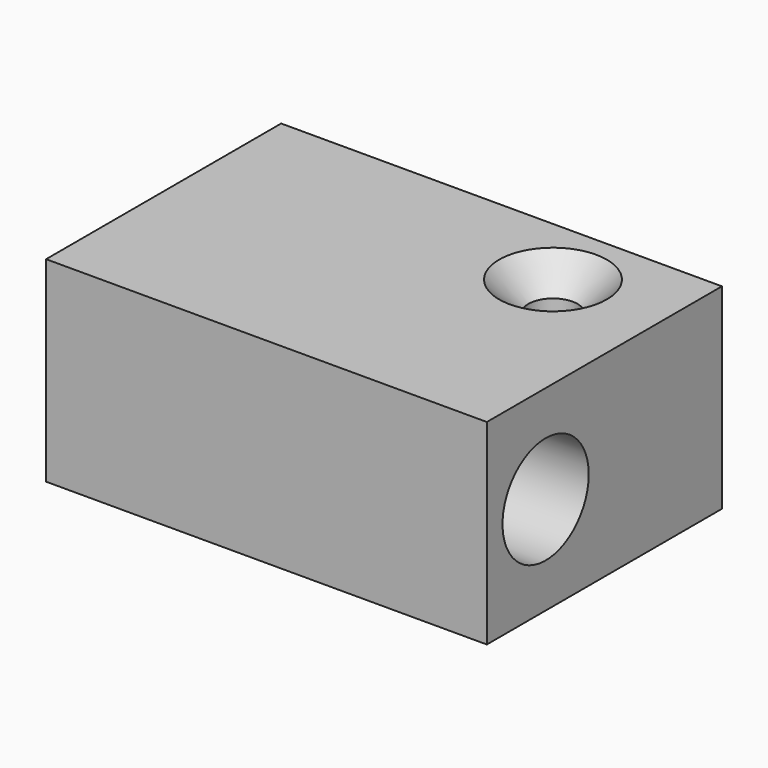
from build123d import *

# Parameters (mm, degrees)
F0_W     = 45
F0_H     = 30
F0_R     = 2.5
F1_DEPTH = 20
F2_R     = 2.5
F3_DEPTH = 45.001
F2_R_2   = 5.5
F4_DEPTH = 20
F5_SIZE  = 2.99999


# Not quite as in the source:
# - a fillet or chamfer is up to 0.001 mm smaller than in the source, because OpenCascade refuses the exact size


with BuildPart() as f1:
    # F0 (on Top) → F1 (new body)
    with BuildSketch(Plane.XY):
        Rectangle(F0_W, F0_H)
        with Locations((11.25, 7.5)):
            Circle(F0_R, mode=Mode.SUBTRACT)
    extrude(amount=F1_DEPTH)

    # F2 (on face) → F3 (cut, through all)
    with BuildSketch(Plane.YZ.offset(22.5)):
        with Locations((-7.5, 10)):
            Circle(F2_R)
    extrude(amount=-F3_DEPTH, mode=Mode.SUBTRACT)

    # F2 (on face) → F4 (cut)
    with BuildSketch(Plane.YZ.offset(22.5)):
        with Locations((-7.5, 10)):
            Circle(F2_R_2)
        with Locations((-7.5, 10)):
            Circle(F2_R, mode=Mode.SUBTRACT)
    extrude(amount=-F4_DEPTH, mode=Mode.SUBTRACT)

    # F5 (size 3 in the source; OpenCascade refuses exactly that, so slightly less here)
    f5_edges = [f1.edges().sort_by_distance(p)[0] for p in [
        (8.75, 7.5, 20),
        (2.5, -13, 10),
    ]]
    chamfer(f5_edges, length=F5_SIZE)


solid = f1.part
